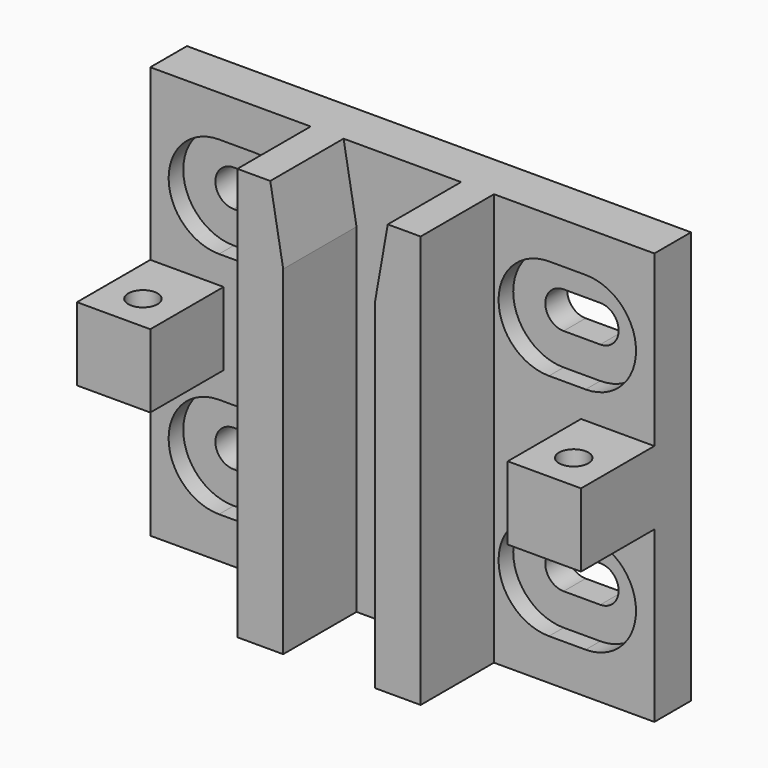
from build123d import *

# Parameters (mm, degrees)
F1_DEPTH   = 45
F3_DEPTH   = 5
F5_DEPTH   = 2
F6_SIZE2   = 1.4106158457
F6_SIZE    = 8
F6_2_SIZE2 = 1.4106158457
F6_2_SIZE  = 8
F7_W       = 8
F7_H       = 8
F8_DEPTH   = 10
F9_R       = 1.6
F10_DEPTH  = 8


# Not quite as in the source:
# - a pattern or mirror of a feature is missing from the dataset's text; its kind, count and spacing are read off the source's solid


with BuildPart() as f1:
    # F0 (on Top) → F1 (new body)
    with BuildSketch(Plane.XY):
        Polygon((-5, -10), (-5, 0), (5, 0), (5, -10), (10, -10), (10, 0), (27.5, 0), (27.5, 5), (-27.5, 5), (-27.5, 0), (-10, 0), (-10, -10), align=None)
    extrude(amount=F1_DEPTH)

    # F2 (on face) → F3 (cut, through all)
    with BuildSketch(Plane.XZ):
        with BuildLine():
            Line((-16, 37), (-20, 37))
            ThreePointArc((-20, 37), (-22, 35), (-20, 33))
            Line((-20, 33), (-16, 33))
            ThreePointArc((-16, 33), (-14, 35), (-16, 37))
        make_face()
        with BuildLine():
            Line((-20, 8), (-16, 8))
            ThreePointArc((-16, 8), (-14, 10), (-16, 12))
            Line((-16, 12), (-20, 12))
            ThreePointArc((-20, 12), (-22, 10), (-20, 8))
        make_face()
    f3 = extrude(amount=-F3_DEPTH, mode=Mode.SUBTRACT)

    # F3_copies: F3 across plane
    add(f3.mirror(Plane(origin=(0, 0, 0), x_dir=(0, 0, 1), z_dir=(1, 0, 0))), mode=Mode.SUBTRACT)

    # F4 (on face) → F5 (cut)
    with BuildSketch(Plane.XZ):
        with BuildLine():
            Line((-16, 40.5), (-20, 40.5))
            ThreePointArc((-20, 40.5), (-25.5, 35), (-20, 29.5))
            Line((-20, 29.5), (-16, 29.5))
            ThreePointArc((-16, 29.5), (-10.5, 35), (-16, 40.5))
        make_face()
        with BuildLine():
            Line((-16, 15.5), (-20, 15.5))
            ThreePointArc((-20, 15.5), (-25.5, 10), (-20, 4.5))
            Line((-20, 4.5), (-16, 4.5))
            ThreePointArc((-16, 4.5), (-10.5, 10), (-16, 15.5))
        make_face()
    f5 = extrude(amount=-F5_DEPTH, mode=Mode.SUBTRACT)

    # F5_copies: F5 across plane
    add(f5.mirror(Plane(origin=(0, 0, 0), x_dir=(0, 0, 1), z_dir=(1, 0, 0))), mode=Mode.SUBTRACT)

    # F6
    f6_edges = [f1.edges().sort_by_distance(p)[0] for p in [
        (-5, -5, 45),
    ]]
    f6_side = f1.faces().sort_by_distance((-5, -5, 22.5))[0]
    chamfer(f6_edges, length=F6_SIZE, length2=F6_SIZE2, reference=f6_side)

    # F6#2
    f6_2_edges = [f1.edges().sort_by_distance(p)[0] for p in [
        (5, -5, 45),
    ]]
    f6_2_side = f1.faces().sort_by_distance((5, -5, 22.5))[0]
    chamfer(f6_2_edges, length=F6_2_SIZE, length2=F6_2_SIZE2, reference=f6_2_side)

    # F7 (on face) → F8 (join)
    with BuildSketch(Plane.XZ):
        with Locations((-23.5, 22.5)):
            Rectangle(F7_W, F7_H)
        with Locations((23.5, 22.5)):
            Rectangle(F7_W, F7_H)
    extrude(amount=F8_DEPTH)

    # F9 (on face) → F10 (cut, through all)
    with BuildSketch(Plane.XY.offset(26.5)):
        with Locations((-23.5, -6)):
            Circle(F9_R)
        with Locations((23.5, -6)):
            Circle(F9_R)
    extrude(amount=-F10_DEPTH, mode=Mode.SUBTRACT)


solid = f1.part
